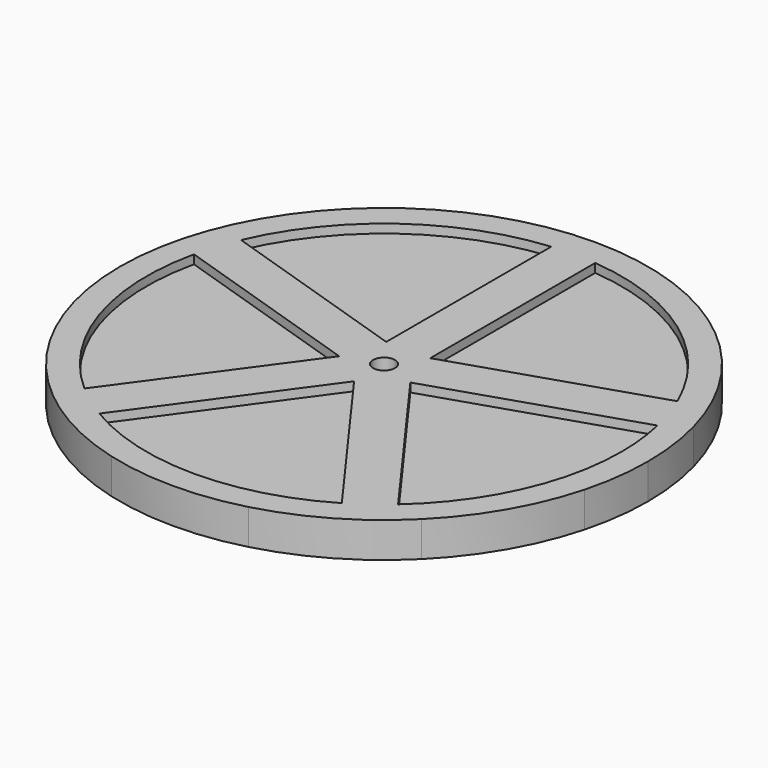
from build123d import *

# Parameters (mm, degrees)
F0_R     = 1.25
F1_DEPTH = 4
F3_DEPTH = 1


with BuildPart() as f1:
    # F0 (on Top) → F1 (new body)
    with BuildSketch(Plane.XY):
        Polygon((20, 0), (28.9777747887, 7.7645713531), (17.3205080757, 10), (21.2132034356, 21.2132034356), (10, 17.3205080757), (7.7645713531, 28.9777747887), (0, 20), (-7.7645713531, 28.9777747887), (-10, 17.3205080757), (-21.2132034356, 21.2132034356), (-17.3205080757, 10), (-28.9777747887, 7.7645713531), (-20, 0), (-28.9777747887, -7.7645713531), (-17.3205080757, -10), (-21.2132034356, -21.2132034356), (-10, -17.3205080757), (-7.7645713531, -28.9777747887), (0, -20), (7.7645713531, -28.9777747887), (10, -17.3205080757), (21.2132034356, -21.2132034356), (17.3205080757, -10), (28.9777747887, -7.7645713531), align=None)
        Circle(F0_R, mode=Mode.SUBTRACT)
        with BuildLine():
            Line((-20, 0), (-28.9777747887, 7.7645713531))
            ThreePointArc((-28.9777747887, 7.7645713531), (-30, 0), (-28.9777747887, -7.7645713531))
            Line((-28.9777747887, -7.7645713531), (-20, 0))
        make_face()
        with BuildLine():
            Line((-17.3205080757, 10), (-21.2132034356, 21.2132034356))
            ThreePointArc((-21.2132034356, 21.2132034356), (-25.9807621135, 15), (-28.9777747887, 7.7645713531))
            Line((-28.9777747887, 7.7645713531), (-17.3205080757, 10))
        make_face()
        with BuildLine():
            Line((-10, 17.3205080757), (-7.7645713531, 28.9777747887))
            ThreePointArc((-7.7645713531, 28.9777747887), (-15, 25.9807621135), (-21.2132034356, 21.2132034356))
            Line((-21.2132034356, 21.2132034356), (-10, 17.3205080757))
        make_face()
        with BuildLine():
            Line((0, 20), (7.7645713531, 28.9777747887))
            ThreePointArc((7.7645713531, 28.9777747887), (0, 30), (-7.7645713531, 28.9777747887))
            Line((-7.7645713531, 28.9777747887), (0, 20))
        make_face()
        with BuildLine():
            Line((10, 17.3205080757), (21.2132034356, 21.2132034356))
            ThreePointArc((21.2132034356, 21.2132034356), (15, 25.9807621135), (7.7645713531, 28.9777747887))
            Line((7.7645713531, 28.9777747887), (10, 17.3205080757))
        make_face()
        with BuildLine():
            Line((17.3205080757, 10), (28.9777747887, 7.7645713531))
            ThreePointArc((28.9777747887, 7.7645713531), (25.9807621135, 15), (21.2132034356, 21.2132034356))
            Line((21.2132034356, 21.2132034356), (17.3205080757, 10))
        make_face()
        with BuildLine():
            ThreePointArc((28.9777747887, -7.7645713531), (29.7433458412, -3.9157857666), (30, 0))
            ThreePointArc((30, 0), (29.7433458412, 3.9157857666), (28.9777747887, 7.7645713531))
            Line((28.9777747887, 7.7645713531), (20, 0))
            Line((20, 0), (28.9777747887, -7.7645713531))
        make_face()
        with BuildLine():
            ThreePointArc((21.2132034356, -21.2132034356), (25.9807621135, -15), (28.9777747887, -7.7645713531))
            Line((28.9777747887, -7.7645713531), (17.3205080757, -10))
            Line((17.3205080757, -10), (21.2132034356, -21.2132034356))
        make_face()
        with BuildLine():
            ThreePointArc((7.7645713531, -28.9777747887), (15, -25.9807621135), (21.2132034356, -21.2132034356))
            Line((21.2132034356, -21.2132034356), (10, -17.3205080757))
            Line((10, -17.3205080757), (7.7645713531, -28.9777747887))
        make_face()
        with BuildLine():
            ThreePointArc((-7.7645713531, -28.9777747887), (0, -30), (7.7645713531, -28.9777747887))
            Line((7.7645713531, -28.9777747887), (0, -20))
            Line((0, -20), (-7.7645713531, -28.9777747887))
        make_face()
        with BuildLine():
            ThreePointArc((-21.2132034356, -21.2132034356), (-15, -25.9807621135), (-7.7645713531, -28.9777747887))
            Line((-7.7645713531, -28.9777747887), (-10, -17.3205080757))
            Line((-10, -17.3205080757), (-21.2132034356, -21.2132034356))
        make_face()
        with BuildLine():
            ThreePointArc((-28.9777747887, -7.7645713531), (-25.9807621135, -15), (-21.2132034356, -21.2132034356))
            Line((-21.2132034356, -21.2132034356), (-17.3205080757, -10))
            Line((-17.3205080757, -10), (-28.9777747887, -7.7645713531))
        make_face()
    extrude(amount=F1_DEPTH)

    # F2 (on face) → F3 (cut)
    with BuildSketch(Plane.XY.offset(4)):
        with BuildLine():
            Line((-24.7956705205, 10.685257294), (-2.5, 3.4409548012))
            Line((-2.5, 3.4409548012), (-2.5, 26.8840101175))
            ThreePointArc((-2.5, 26.8840101175), (-15.8702018119, 21.8434588481), (-24.7956705205, 10.685257294))
        make_face()
        with BuildLine():
            Line((2.5, 26.8840101175), (2.5, 3.4409548012))
            Line((2.5, 3.4409548012), (24.7956705205, 10.685257294))
            ThreePointArc((24.7956705205, 10.685257294), (15.8702018119, 21.8434588481), (2.5, 26.8840101175))
        make_face()
        with BuildLine():
            Line((26.3407554924, 5.9299747125), (4.0450849719, -1.3143277803))
            Line((4.0450849719, -1.3143277803), (17.8245671555, -20.2801579313))
            ThreePointArc((17.8245671555, -20.2801579313), (24.5994239079, -11.1296155999), (27, 0))
            ThreePointArc((27, 0), (26.8346827659, 2.9832534007), (26.3407554924, 5.9299747125))
        make_face()
        with BuildLine():
            Line((13.7794821836, -23.2190841928), (0, -4.2532540418))
            Line((0, -4.2532540418), (-13.7794821836, -23.2190841928))
            ThreePointArc((-13.7794821836, -23.2190841928), (0, -27), (13.7794821836, -23.2190841928))
        make_face()
        with BuildLine():
            Line((-17.8245671555, -20.2801579313), (-4.0450849719, -1.3143277803))
            Line((-4.0450849719, -1.3143277803), (-26.3407554924, 5.9299747125))
            ThreePointArc((-26.3407554924, 5.9299747125), (-25.67852594, -8.3434588481), (-17.8245671555, -20.2801579313))
        make_face()
    extrude(amount=-F3_DEPTH, mode=Mode.SUBTRACT)


solid = f1.part
